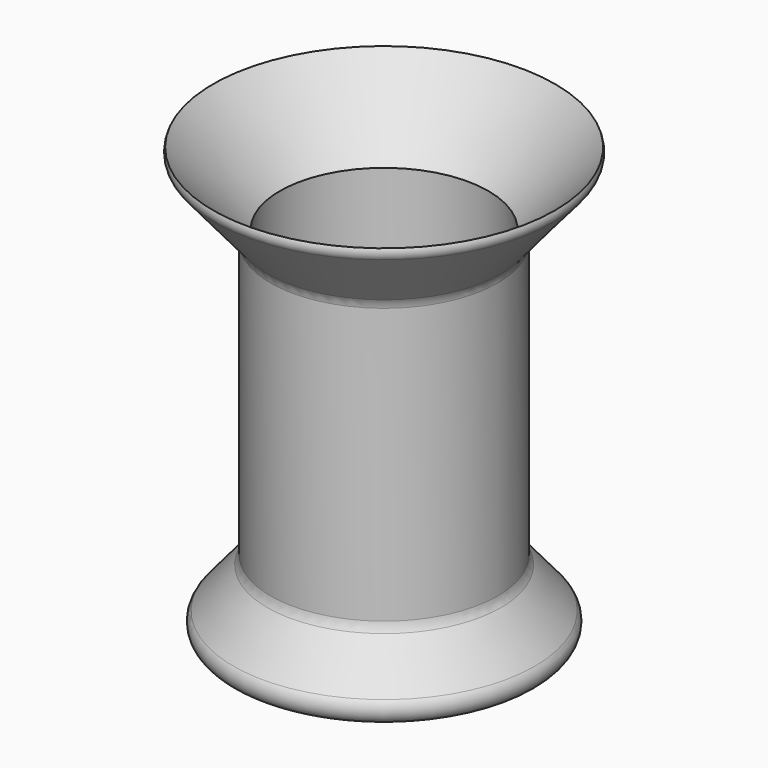
from build123d import *

# Parameters (mm, degrees)
F2_R = 2


# Not quite as in the source:
# - a fillet or chamfer that OpenCascade refuses, or shapes differently, is made with other operations: its cross-section is extruded or revolved along the edge and cut away or added


with BuildPart() as f1:
    # F0 (on Front) → F1 (revolve)
    with BuildSketch(Plane.XZ):
        Polygon((15.8820929868, -20), (15.8820929868, 0), (15.8820929868, 20), (25, 30.8662984399), (23.9358222275, 30.8662984399), (14.5927630612, 20.7279404685), (14.5927630612, 0.3639702343), (14.5927630612, -20), (21.0905159717, -28.2129982056), (2.4876487441, -28.2129982056), (2.4876487441, -29.5023282056), (22.5661631538, -29.5023282056), (23.8554930795, -29.5023282056), align=None)
    revolve(axis=Axis((0, 0, 0), (0, 0, -1)))

    # F2
    f2_edges = [f1.edges().sort_by_distance(p)[0] for p in [
        (-15.882093, 0, -20),
        (-15.882093, 0, 20),
        (-23.855493, 0, -29.502328),
    ]]
    fillet(f2_edges, radius=F2_R)

    # F3: fillet of radius 1.5 on 1 edges, made by hand

    # F3_s1 → F3_t2 (revolve, cut)
    with BuildSketch(Plane.XZ):
        with BuildLine():
            ThreePointArc((23.7026404335, 29.319932157), (24.0367869093, 30.060330686), (23.9359604662, 30.8663566642))
            Line((23.9359604662, 30.8663566642), (23.9636082001, 30.878001526))
            ThreePointArc((23.9636082001, 30.878001526), (24.4679802331, 30.8962984399), (25, 30.8962984399))
            Line((25, 30.8962984399), (25.0229813333, 30.8470148116))
            ThreePointArc((25.0229813333, 30.8470148116), (24.3742440967, 30.0738798792), (23.7256217668, 29.3006485287))
            Line((23.7256217668, 29.3006485287), (23.7026404335, 29.319932157))
        make_face()
    revolve(axis=Axis((0, 0, 30.8662984399), (0, 0, -1)), mode=Mode.SUBTRACT)


solid = f1.part
